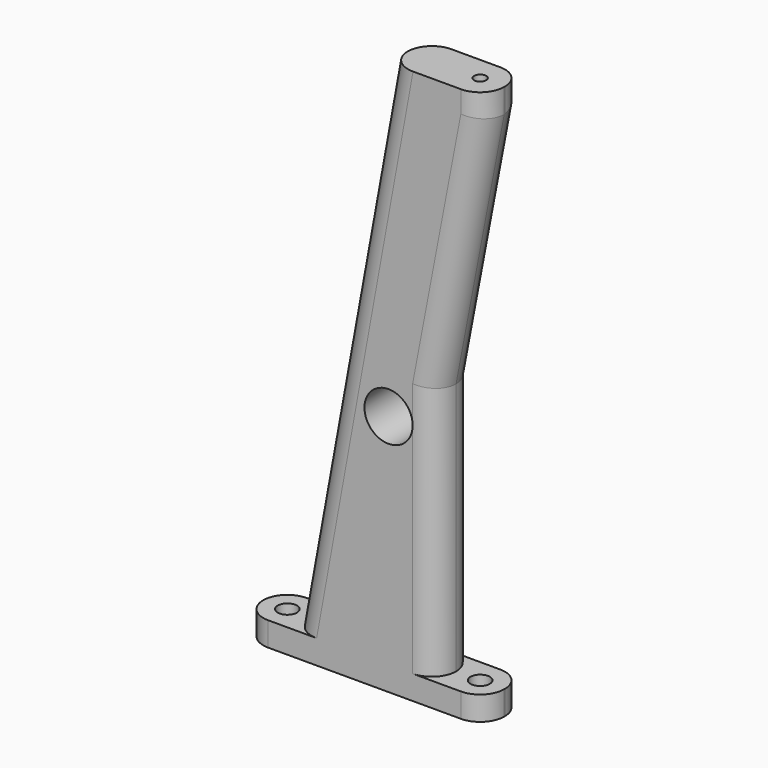
from build123d import *

# Parameters (mm, degrees)
F1_DEPTH     = 10
F2_R         = 2
F3_DEPTH     = 115.001
F4_R         = 2
F4_R_2       = 1.25
F5_DEPTH     = 5
F6_R         = 2
F7_DEPTH     = 5
F9_DEPTH     = 10
F10_R        = 4.99999
F11_R        = 5
F12_DEPTH    = 10.001
F14_DEPTH    = 10
F15_T4_DEPTH = 78.4438958161
F15_T9_DEPTH = 78.4438958161
F16_R        = 4.99999


# Not quite as in the source:
# - a fillet or chamfer that OpenCascade refuses, or shapes differently, is made with other operations: its cross-section is extruded or revolved along the edge and cut away or added
# - a fillet or chamfer is up to 0.001 mm smaller than in the source, because OpenCascade refuses the exact size


with BuildPart() as f1:
    # F0 (on Front) → F1 (new body)
    with BuildSketch(Plane.XZ):
        Polygon((0, 115), (0, 0), (10, 0), (20, 0), (20, 5), (10, 5), (10, 110), (20, 110), (20, 115), (10, 115), align=None)
    extrude(amount=F1_DEPTH)

    # F2 (on face) → F3 (cut, through all)
    with BuildSketch(Plane.XY.offset(115)):
        with BuildLine():
            Line((0, -10), (5, -10))
            ThreePointArc((5, -10), (1.4644660941, -8.5355339059), (0, -5))
            Line((0, -5), (0, -10))
        make_face()
        with BuildLine():
            Line((0, 0), (0, -5))
            ThreePointArc((0, -5), (1.4644660941, -1.4644660941), (5, 0))
            Line((5, 0), (0, 0))
        make_face()
        with BuildLine():
            ThreePointArc((15.2, 0), (18.5941125497, -1.4058874503), (20, -4.8))
            Line((20, -4.8), (20, 0))
            Line((20, 0), (15.2, 0))
        make_face()
        with BuildLine():
            ThreePointArc((20, -5), (18.5355339059, -8.5355339059), (15, -10))
            Line((15, -10), (20, -10))
            Line((20, -10), (20, -5))
        make_face()
        with Locations((15, -5)):
            Circle(F2_R)
    extrude(amount=-F3_DEPTH, mode=Mode.SUBTRACT)

    # F4 (on face) → F5 (join)
    with BuildSketch(Plane.XY.offset(115)):
        with Locations((15, -5)):
            Circle(F4_R)
        with Locations((15, -5)):
            Circle(F4_R_2, mode=Mode.SUBTRACT)
    extrude(amount=-F5_DEPTH)

    # F6 (on face) → F7 (join)
    with BuildSketch(Plane(origin=(0, 0, 0), x_dir=(1, 0, 0), z_dir=(0, 0, -1))):
        with BuildLine():
            Line((-25, 0), (5, 0))
            ThreePointArc((5, 0), (0, 5), (5, 10))
            Line((5, 10), (-25, 10))
            ThreePointArc((-25, 10), (-28.5355339059, 8.5355339059), (-30, 5))
            ThreePointArc((-30, 5), (-28.5355339059, 1.4644660941), (-25, 0))
        make_face()
        with Locations((-25, 5)):
            Circle(F6_R, mode=Mode.SUBTRACT)
    extrude(amount=-F7_DEPTH)

    # F8 (on face) → F9 (join)
    with BuildSketch(Plane.XZ.offset(10)):
        Polygon((0, 115), (-20, 5), (5, 5), (5, 115), align=None)
    extrude(amount=-F9_DEPTH)

    # F10 (radius 5 in the source; OpenCascade refuses exactly that, so slightly less here)
    f10_edges = [f1.edges().sort_by_distance(p)[0] for p in [
        (-10, 0, 60),
        (-10, -10, 60),
    ]]
    fillet(f10_edges, radius=F10_R)

    # F11 (on face) → F12 (cut, through all)
    with BuildSketch(Plane.XZ.offset(10)):
        with Locations((0, 50.3422953188)):
            Circle(F11_R)
    extrude(amount=-F12_DEPTH, mode=Mode.SUBTRACT)

    # F13 (on face) → F14 (join)
    with BuildSketch(Plane(origin=(0, 0, 0), x_dir=(-1, 0, 0), z_dir=(0, 1, 0))):
        Polygon((-20, 110), (-10, 57.5), (-10, 110), (-15.2, 110), align=None)
    extrude(amount=-F14_DEPTH)

    # F15: fillet of radius 5 on 2 edges, made by hand


with BuildPart() as f15_tool2:
    # F15_s3 → F15_t4 (new body)
    with BuildSketch(Plane(origin=(23.2579385477, 0, 122.1041773757), x_dir=(0, 1, 0), z_dir=(-0.1871121079, 0, -0.9823385664))):
        with BuildLine():
            ThreePointArc((0, -5.9355605394), (-1.4644660941, -2.4000266335), (-5, -0.9355605394))
            Line((-5, -0.9355605394), (0, -0.9355605394))
            Line((0, -0.9355605394), (0, -5.9355605394))
        make_face()
    extrude(amount=F15_T4_DEPTH)

    split(bisect_by=Plane.YZ.offset(10), keep=Keep.TOP)


with BuildPart() as f1_1:
    add(f1.part)

    # F15_t1: cut F15_tool2
    add(f15_tool2.part, mode=Mode.SUBTRACT)


with BuildPart() as f15_tool7:
    # F15_s8 → F15_t9 (new body)
    with BuildSketch(Plane(origin=(23.2579385477, 0, 122.1041773757), x_dir=(0, 1, 0), z_dir=(-0.1871121079, 0, -0.9823385664))):
        with BuildLine():
            ThreePointArc((-10, -5.9355605394), (-8.5355339059, -2.4000266335), (-5, -0.9355605394))
            Line((-5, -0.9355605394), (-10, -0.9355605394))
            Line((-10, -0.9355605394), (-10, -5.9355605394))
        make_face()
    extrude(amount=F15_T9_DEPTH)

    split(bisect_by=Plane.YZ.offset(10), keep=Keep.TOP)


with BuildPart() as f1_2:
    add(f1_1.part)

    # F15_t6: cut F15_tool7
    add(f15_tool7.part, mode=Mode.SUBTRACT)

    # F16 (radius 5 in the source; OpenCascade refuses exactly that, so slightly less here)
    f16_edges = [f1_2.edges().sort_by_distance(p)[0] for p in [
        (10, 0, 44.610974),
        (10, -10, 44.610974),
    ]]
    fillet(f16_edges, radius=F16_R)


solid = f1_2.part
